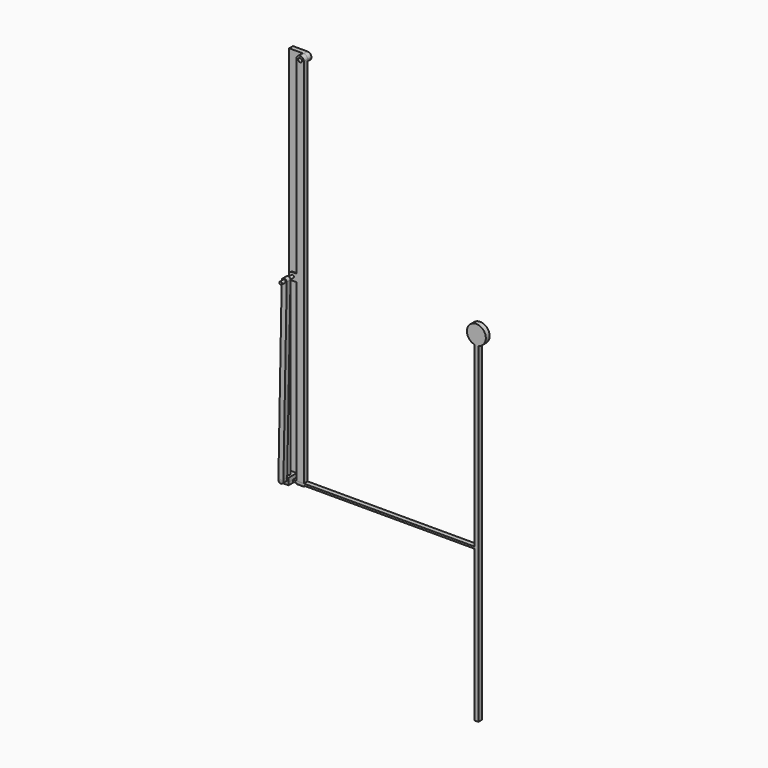
from build123d import *

# Parameters (mm, degrees)
F0_R      = 10
F1_DEPTH  = 25
F2_R      = 10
F3_DEPTH  = 25
F4_W      = 40
F4_H      = 15
F5_DEPTH  = 55
F6_W      = 4
F6_H      = 40
F7_DEPTH  = 40
F9_DEPTH  = 5
F10_R     = 7.5
F11_DEPTH = 919
F12_DEPTH = 20
F14_R     = 5
F14_R_2   = 7.5
F15_DEPTH = 25
F13_R     = 5
F16_DEPTH = 25
F8_R      = 7.5
F17_DEPTH = 78.3
F18_W     = 1000
F18_H     = 10
F18_W_2   = 20
F18_H_2   = 800
F19_DEPTH = 25


with BuildPart() as f1:
    # F0 (on Front) → F1 (new body)
    with BuildSketch(Plane.XZ):
        Polygon((20, 960), (20, 1000), (-20, 1000), (-20, -1000), (20, -1000), align=None)
        with BuildLine():
            Line((57.5, 1000), (20, 1000))
            Line((20, 1000), (20, 960))
            Line((20, 960), (57.5, 960))
            ThreePointArc((57.5, 960), (37.5, 980), (57.5, 1000))
        make_face()
        with BuildLine():
            ThreePointArc((77.5, 980), (71.6421356237, 994.1421356237), (57.5, 1000))
            ThreePointArc((57.5, 1000), (37.5, 980), (57.5, 960))
            ThreePointArc((57.5, 960), (71.6421356237, 965.8578643763), (77.5, 980))
        make_face()
        with Locations((57.5, 980)):
            Circle(F0_R, mode=Mode.SUBTRACT)
    extrude(amount=F1_DEPTH)

    # F4 (on face) → F5 (join)
    with BuildSketch(Plane.XZ.offset(25)):
        with Locations((0, -992.5)):
            Rectangle(F4_W, F4_H)
    extrude(amount=F5_DEPTH)

    # F10 (on face) → F11 (join)
    with BuildSketch(Plane.XY.offset(-985)):
        with Locations((0, -52.5)):
            Circle(F10_R)
    extrude(amount=F11_DEPTH)


with BuildPart() as f3:
    # F2 (on face) → F3 (new body)
    with BuildSketch(Plane.XZ.offset(25)):
        with BuildLine():
            Line((77.5, -1000), (77.5, 980))
            ThreePointArc((77.5, 980), (71.6421356237, 965.8578643763), (57.5, 960))
            Line((57.5, 960), (37.5, 960))
            Line((37.5, 960), (37.5, -1000))
            Line((37.5, -1000), (77.5, -1000))
        make_face()
        with BuildLine():
            ThreePointArc((77.5, 980), (71.6421356237, 994.1421356237), (57.5, 1000))
            ThreePointArc((57.5, 1000), (43.3578643763, 994.1421356237), (37.5, 980))
            ThreePointArc((37.5, 980), (43.3578643763, 965.8578643763), (57.5, 960))
            ThreePointArc((57.5, 960), (71.6421356237, 965.8578643763), (77.5, 980))
        make_face()
        with Locations((57.5, 980)):
            Circle(F2_R, mode=Mode.SUBTRACT)
        with BuildLine():
            ThreePointArc((57.5, 960), (43.3578643763, 965.8578643763), (37.5, 980))
            Line((37.5, 980), (37.5, 960))
            Line((37.5, 960), (57.5, 960))
        make_face()
    extrude(amount=F3_DEPTH)

    # F6 (on face) → F7 (join)
    with BuildSketch(Plane(origin=(37.5, 0, 0), x_dir=(0, -1, 0), z_dir=(-1, 0, 0))):
        with Locations((48, -40)):
            Rectangle(F6_W, F6_H)
    extrude(amount=F7_DEPTH)

    # F8 (on face) → F9 (cut)
    with BuildSketch(Plane.XZ.offset(50)):
        with BuildLine():
            ThreePointArc((-2.5, -40), (3.3578643763, -25.8578643763), (17.5, -20))
            Line((17.5, -20), (-2.5, -20))
            Line((-2.5, -20), (-2.5, -40))
        make_face()
        with BuildLine():
            Line((-2.5, -60), (17.5, -60))
            ThreePointArc((17.5, -60), (3.3578643763, -54.1421356237), (-2.5, -40))
            Line((-2.5, -40), (-2.5, -60))
        make_face()
    extrude(amount=-F9_DEPTH, mode=Mode.SUBTRACT)

    # F8 (on face) → F17 (join)
    with BuildSketch(Plane.XZ.offset(50)):
        with Locations((17.5, -40)):
            Circle(F8_R)
    extrude(amount=F17_DEPTH)


with BuildPart() as f12:
    # F12 (new): a face of the model
    f12_faces = [f1.part.faces().sort_by_distance(p)[0] for p in [
        (19.3199264746, -52.5, -985),
    ]]
    extrude(f12_faces, amount=F12_DEPTH)

    # F13 (on face) → F16 (join)
    with BuildSketch(Plane.XZ.offset(80)):
        with Locations((0, -975)):
            Circle(F13_R)
    extrude(amount=F16_DEPTH)


with BuildPart() as f15:
    # F14 (on face) → F15 (new body)
    with BuildSketch(Plane.XZ.offset(80)):
        with BuildLine():
            Line((-8.6838635851, -965), (8.6838635851, -965))
            ThreePointArc((8.6838635851, -965), (0, -961.755775343), (-8.6838635851, -965))
        make_face()
        with BuildLine():
            Line((13.2419054738, -975.2478430705), (13.4337100232, -965))
            Line((13.4337100232, -965), (8.6838635851, -965))
            ThreePointArc((8.6838635851, -965), (12.0503221321, -969.5046180045), (13.244224657, -975))
            ThreePointArc((13.244224657, -975), (13.2436448485, -975.1239269605), (13.2419054738, -975.2478430705))
        make_face()
        with BuildLine():
            Line((-8.6838635851, -965), (-13.0593784724, -965))
            Line((-13.0593784724, -965), (-13.2419052476, -974.7521448442))
            ThreePointArc((-13.2419052476, -974.7521448442), (-11.9983714308, -969.3920975603), (-8.6838635851, -965))
        make_face()
        with BuildLine():
            ThreePointArc((-0.2478435243, -988.2419054653), (4.5187494263, -987.4495136606), (8.6838635851, -985))
            Line((8.6838635851, -985), (-8.6838635851, -985))
            ThreePointArc((-8.6838635851, -985), (-4.7509299861, -987.3627727889), (-0.2478435243, -988.2419054653))
        make_face()
        with BuildLine():
            Line((13.4337100232, -965), (30.7419054788, -40.2478428035))
            ThreePointArc((30.7419054788, -40.2478428035), (17.2521509276, -53.2419053614), (4.2580947559, -39.7521446587))
            Line((4.2580947559, -39.7521446587), (-13.0593784724, -965))
            Line((-13.0593784724, -965), (-8.6838635851, -965))
            ThreePointArc((-8.6838635851, -965), (0, -961.755775343), (8.6838635851, -965))
            Line((8.6838635851, -965), (13.4337100232, -965))
        make_face()
        with BuildLine():
            ThreePointArc((8.6838635851, -985), (11.9983739898, -980.6078969645), (13.2419054738, -975.2478430705))
            ThreePointArc((13.2419054738, -975.2478430705), (13.2436448485, -975.1239269605), (13.244224657, -975))
            ThreePointArc((13.244224657, -975), (12.0503221321, -969.5046180045), (8.6838635851, -965))
            Line((8.6838635851, -965), (-8.6838635851, -965))
            ThreePointArc((-8.6838635851, -965), (-11.9983714308, -969.3920975603), (-13.2419052476, -974.7521448442))
            ThreePointArc((-13.2419052476, -974.7521448442), (-12.1012176474, -980.3823803484), (-8.6838635851, -985))
            Line((-8.6838635851, -985), (8.6838635851, -985))
        make_face()
        with Locations((0, -975)):
            Circle(F14_R, mode=Mode.SUBTRACT)
        with BuildLine():
            ThreePointArc((4.2580947559, -39.7521446587), (17.2521509276, -53.2419053614), (30.7419054788, -40.2478428035))
            ThreePointArc((30.7419054788, -40.2478428035), (30.7436448497, -40.1239268271), (30.744224657, -40))
            ThreePointArc((30.744224657, -40), (26.9523000332, -30.7229578611), (17.7478412406, -26.758094492))
            ThreePointArc((17.7478412406, -26.758094492), (8.31181412, -30.4613037055), (4.2580947559, -39.7521446587))
        make_face()
        with Locations((17.5, -40)):
            Circle(F14_R_2, mode=Mode.SUBTRACT)
    extrude(amount=F15_DEPTH)


with BuildPart() as f1_1:
    add(f1.part)

    # F18 (on face) → F19 (join)
    with BuildSketch(Plane.XZ.offset(25)):
        with Locations((480, -990)):
            Rectangle(F18_W, F18_H)
        with Locations((990, -990)):
            Rectangle(F18_W_2, F18_H)
        with BuildLine():
            Line((980, -43.9897948557), (980, -985))
            Line((980, -985), (1000, -985))
            Line((1000, -985), (1000, -43.9897948557))
            ThreePointArc((1000, -43.9897948557), (990, -45), (980, -43.9897948557))
        make_face()
        with Locations((990, -1395)):
            Rectangle(F18_W_2, F18_H_2)
        with BuildLine():
            ThreePointArc((1040, 5), (958.3772233983, 43.7298334621), (980, -43.9897948557))
            Line((980, -43.9897948557), (980, 5))
            Line((980, 5), (1000, 5))
            Line((1000, 5), (1000, -43.9897948557))
            ThreePointArc((1000, -43.9897948557), (1028.7298334621, -26.6227766017), (1040, 5))
        make_face()
        with BuildLine():
            Line((980, 5), (980, -43.9897948557))
            ThreePointArc((980, -43.9897948557), (990, -45), (1000, -43.9897948557))
            Line((1000, -43.9897948557), (1000, 5))
            Line((1000, 5), (980, 5))
        make_face()
    extrude(amount=F19_DEPTH)


solid = Compound([f3.part, f12.part, f15.part, f1_1.part])
